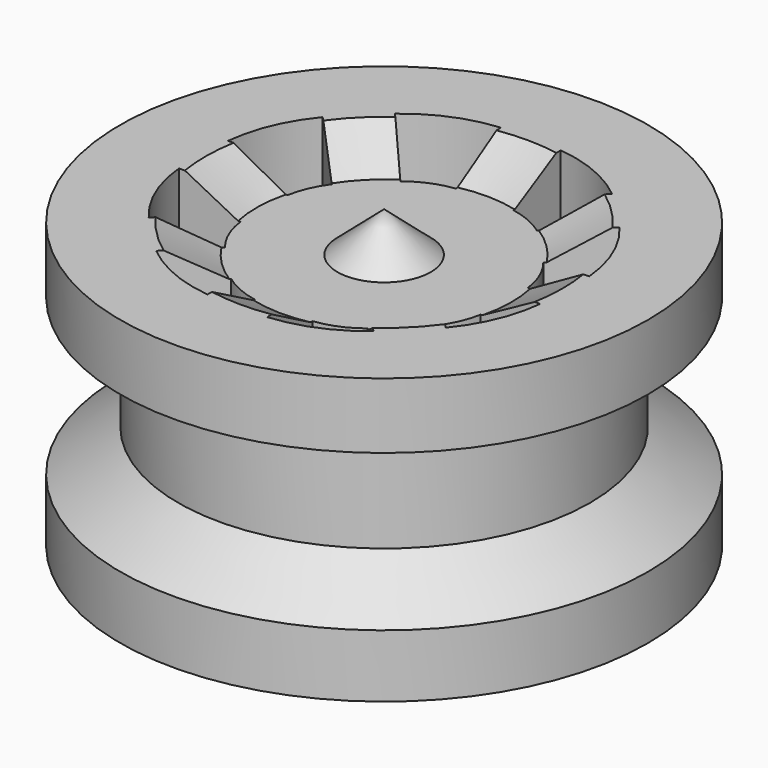
from build123d import *

# Parameters (mm, degrees)
F3_DEPTH        = 127
F3_COPIES_COUNT = 4


# Not quite as in the source:
# - ends of sketch curves that miss each other by under 0.0002 mm in the source are joined
# - a pattern or mirror of a feature is missing from the dataset's text; its kind, count and spacing are read off the source's solid
# - a feature names something its author has since deleted; it is built from what else it names


with BuildPart() as f1:
    # F0 (on Front) → F1 (revolve)
    with BuildSketch(Plane.XZ):
        Polygon((0, 35.4743129574), (0, 0), (4.6190516926, 4.819879774), (15.2308195829, 4.819879774), (22.1714451909, 0), (24.8705781996, 0), (31.6184088588, 0), (31.6184088588, 7.5190118514), (24.6777832508, 12.5316865742), (24.6777832508, 22.7498319), (31.6184088588, 26.220144704), (31.6184088588, 34.0789705515), (21.3958136737, 34.0789705515), (15.2910613324, 30.654432252), (5.5910609663, 30.654432252), align=None)
    revolve(axis=Axis((0, 0, 17.7371564787), (0, 0, -1)))

    # F2 (on Top) → F3 (cut)
    with BuildSketch(Plane.XY):
        with BuildLine():
            Line((-8.115033377, -12.7501504258), (-13.0466232076, -17.822753638))
            ThreePointArc((-13.0466232076, -17.822753638), (-8.7024720698, -20.4552886114), (-3.7824651226, -21.7183884233))
            Line((-3.7824651226, -21.7183884233), (-3.8017209154, -14.6126616746))
            ThreePointArc((-3.8017209154, -14.6126616746), (-6.0656566611, -13.9298502242), (-8.115033377, -12.7501504258))
        make_face()
        with BuildLine():
            Line((-14.6720074117, -3.1553390436), (-21.8130666763, -3.460330423))
            ThreePointArc((-21.8130666763, -3.460330423), (-20.5603310713, -8.5289225119), (-17.8181231022, -12.9719246179))
            Line((-17.8181231022, -12.9719246179), (-12.5861142183, -8.1048054074))
            ThreePointArc((-12.5861142183, -8.1048054074), (-13.9770302322, -5.7767197599), (-14.6720074117, -3.1553390436))
        make_face()
    f3 = extrude(amount=F3_DEPTH, mode=Mode.SUBTRACT)

    # F3_copies: F3 ×4 about axis
    f3_copies_axis = Axis((0, 0, 0), (0, 0, 1))
    for i in range(1, F3_COPIES_COUNT):
        add(f3.rotate(f3_copies_axis, i * 360 / F3_COPIES_COUNT), mode=Mode.SUBTRACT)


solid = f1.part
